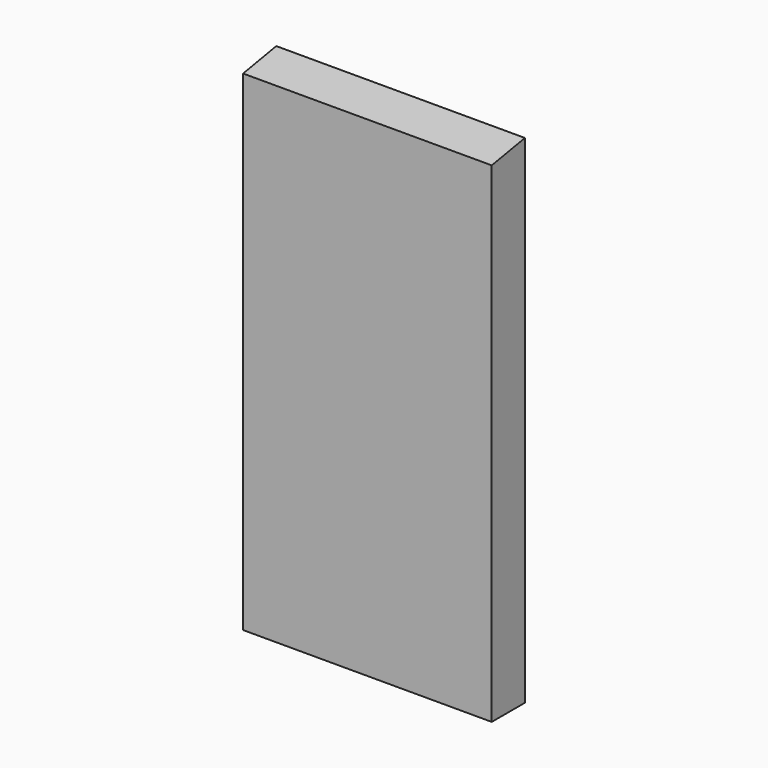
from build123d import *

# Parameters (mm, degrees)
F0_W     = 152.4
F0_H     = 304.8
F1_DEPTH = 25.4
F2_SIZE2 = 4.478695
F2_SIZE  = 25.39999


# Not quite as in the source:
# - a fillet or chamfer is up to 0.001 mm smaller than in the source, because OpenCascade refuses the exact size


with BuildPart() as f1:
    # F0 (on Front) → F1 (new body)
    with BuildSketch(Plane.XZ):
        with Locations((-1.5368815511, 26.1107931341)):
            Rectangle(F0_W, F0_H)
    extrude(amount=F1_DEPTH)

    # F2 (size 25.4 and 4.47870531 in the source; OpenCascade refuses exactly that, so slightly less here)
    f2_edges = [f1.edges().sort_by_distance(p)[0] for p in [
        (-1.536882, -25.4, 178.510793),
    ]]
    f2_side = f1.faces().sort_by_distance((-1.536882, -12.7, 178.510793))[0]
    chamfer(f2_edges, length=F2_SIZE, length2=F2_SIZE2, reference=f2_side)


solid = f1.part
